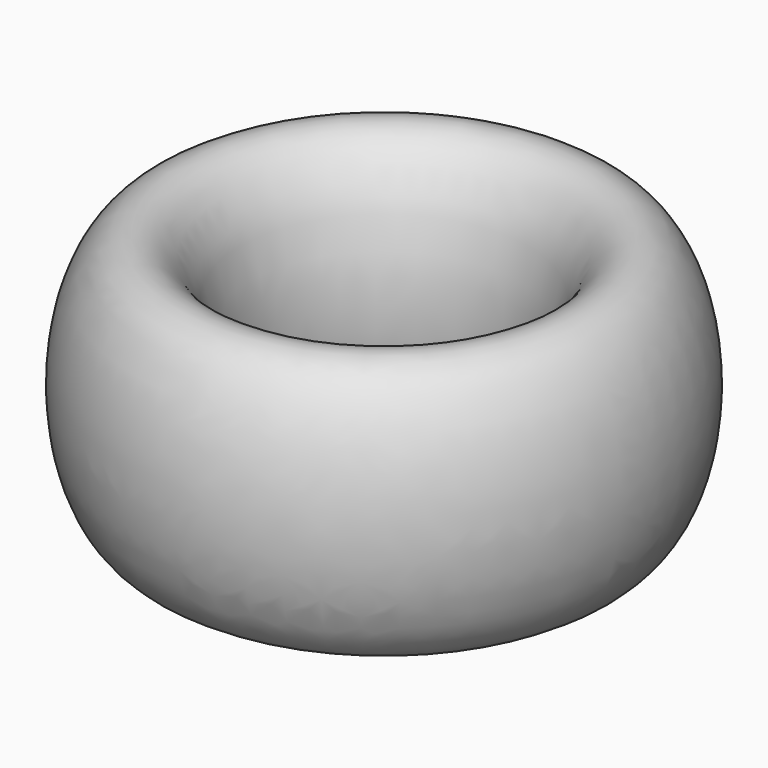
from build123d import *


# Not quite as in the source:
# - a feature names something its author has since deleted; it is built from what else it names


with BuildPart() as f1:
    # F0 (on Front) → F1 (revolve)
    with BuildSketch(Plane.XZ):
        with BuildLine():
            Line((0, 0), (37.5, 0))
            add(Edge.make_bspline(
                [(37.5, 0), (53.554286417, 0), (49.6185611819, 31.1287763481), (45.6828359468, 62.2575526962), (31.5582439085, 46.995048038), (17.4336518702, 31.7325433799), (28.2946943541, 8.0870052367)],
                knots=[3.1415926536, 3.1415926536, 3.1415926536, 4.9600644783, 4.9600644783, 6.778536303, 6.778536303, 8.5970081277, 8.5970081277, 8.5970081277], degree=2, weights=[1, 0.6143488203, 1, 0.6143488203, 1, 0.6143488203, 1]))
            ThreePointArc((28.2946943541, 8.0870052367), (27.9603000834, 3.3013916719), (23.7510824493, 1))
            Line((23.7510824493, 1), (0, 1))
            Line((0, 1), (0, 0))
        make_face()
    revolve(axis=Axis((0, 0, 50), (0, 0, 1)))


solid = f1.part
